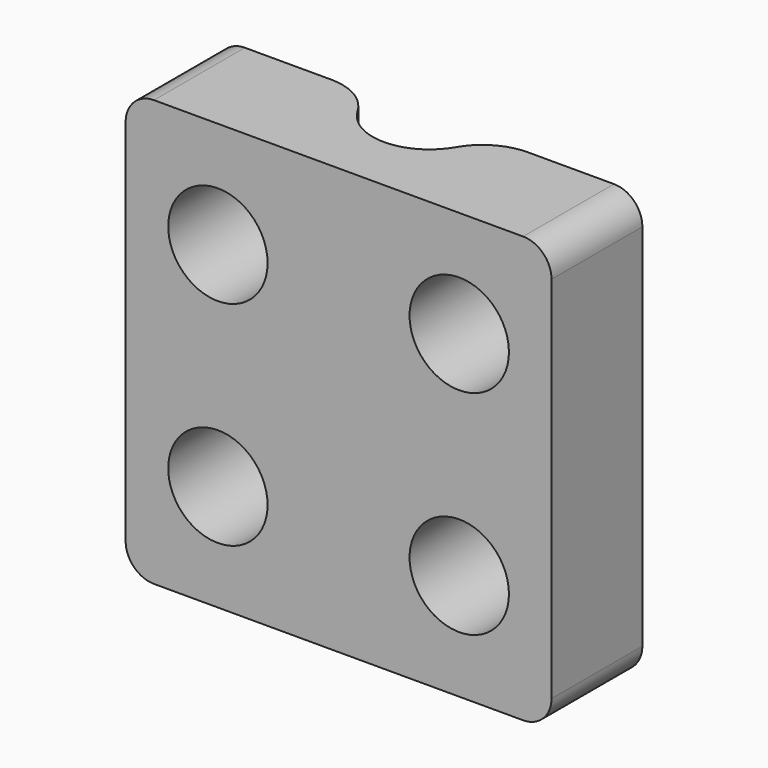
from build123d import *

# Parameters (mm, degrees)
F0_W         = 15
F0_H         = 8
F2_DEPTH     = 15
F1_R         = 2
F3_DEPTH     = 20
F4_R         = 1.75
F5_DEPTH     = 15
F6_DEPTH     = 25
F8_R         = 1.75
F9_DEPTH     = 25
F10_R        = 1.75
F11_DEPTH    = 25
F7_W         = 19.053414464
F7_H         = 8.769848384
F12_DEPTH    = 25
F13_T1_DEPTH = 22.3205080757
F14_R        = 1


# Not quite as in the source:
# - a fillet or chamfer that OpenCascade refuses, or shapes differently, is made with other operations: its cross-section is extruded or revolved along the edge and cut away or added


with BuildPart() as f2:
    # F0 (on Top) → F2 (new body)
    with BuildSketch(Plane.XY):
        Rectangle(F0_W, F0_H)
    extrude(amount=F2_DEPTH)

    # F1 (on Top) → F3 (cut)
    with BuildSketch(Plane.XY):
        Circle(F1_R)
    extrude(amount=F3_DEPTH, mode=Mode.SUBTRACT)

    # F4 (on Front) → F5 (cut)
    with BuildSketch(Plane.XZ):
        with Locations((-4.25, 11.25)):
            Circle(F4_R)
    extrude(amount=F5_DEPTH, mode=Mode.SUBTRACT)

    # F4 (on Front) → F6 (cut)
    with BuildSketch(Plane.XZ):
        with Locations((-4.25, 11.25)):
            Circle(F4_R)
    extrude(amount=-F6_DEPTH, mode=Mode.SUBTRACT)

    # F8 (on face) → F9 (cut)
    with BuildSketch(Plane.XZ.offset(4)):
        with Locations((-4.25, 3.75)):
            Circle(F8_R)
    extrude(amount=-F9_DEPTH, mode=Mode.SUBTRACT)

    # F10 (on face) → F11 (cut)
    with BuildSketch(Plane.XZ.offset(4)):
        with Locations((4.25, 11.25)):
            Circle(F10_R)
        with Locations((4.25, 3.75)):
            Circle(F10_R)
    extrude(amount=-F11_DEPTH, mode=Mode.SUBTRACT)

    # F7 (on Top) → F12 (cut)
    with BuildSketch(Plane.XY):
        with Locations((0, 4.384924192)):
            Rectangle(F7_W, F7_H)
    extrude(amount=F12_DEPTH, mode=Mode.SUBTRACT)

    # F13: fillet of radius 2 on 2 edges, made by hand

    # F13_s2 → F13_t1 (cut)
    with BuildSketch(Plane.XY.offset(-3.6602540378)):
        with BuildLine():
            ThreePointArc((1.7320508076, -1), (2.4641016151, -0.2679491924), (3.4641016151, 0))
            Line((3.4641016151, 0), (2, 0))
            ThreePointArc((2, 0), (1.9318516526, -0.5176380902), (1.7320508076, -1))
        make_face()
        with BuildLine():
            ThreePointArc((-3.4641016151, 0), (-2.4641016151, -0.2679491924), (-1.7320508076, -1))
            ThreePointArc((-1.7320508076, -1), (-1.9318516526, -0.5176380902), (-2, 0))
            Line((-2, 0), (-3.4641016151, 0))
        make_face()
    extrude(amount=F13_T1_DEPTH, mode=Mode.SUBTRACT)

    # F14
    f14_edges = [f2.edges().sort_by_distance(p)[0] for p in [
        (-7.5, -2, 15),
        (-7.5, -2, 0),
        (7.5, -2, 15),
        (7.5, -2, 0),
    ]]
    fillet(f14_edges, radius=F14_R)


solid = f2.part
